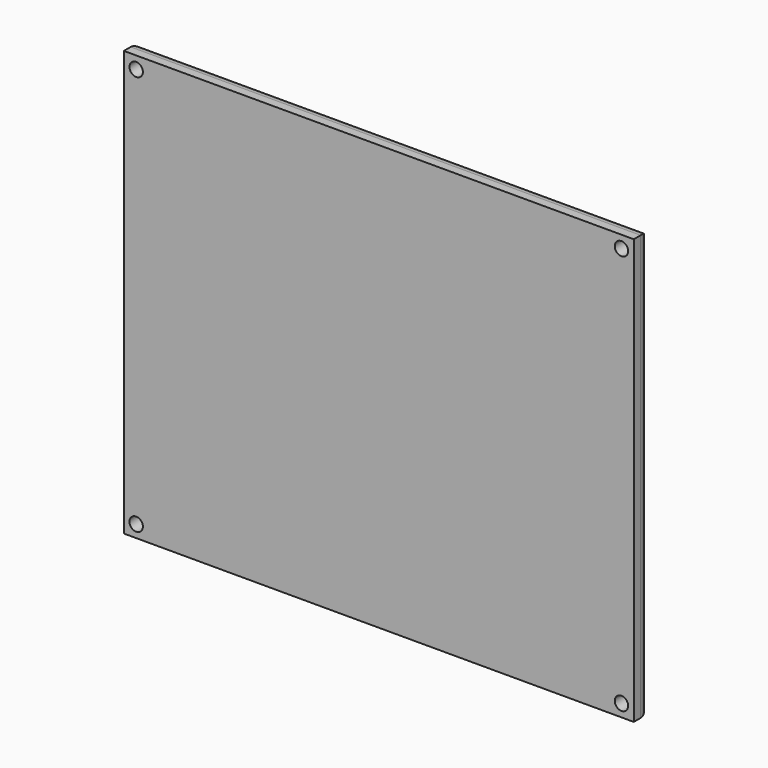
from build123d import *

# Parameters (mm, degrees)
F0_W           = 120
F0_H           = 100
F1_DEPTH       = 5
F2_D           = 3.15
F2_CSINK_D     = 5
F2_CSINK_ANGLE = 90
F3_T1_DEPTH    = 135
F3_T3_DEPTH    = 115


# Not quite as in the source:
# - a fillet or chamfer that OpenCascade refuses, or shapes differently, is made with other operations: its cross-section is extruded or revolved along the edge and cut away or added


with BuildPart() as f1:
    # F0 (on Front) → F1 (new body)
    with BuildSketch(Plane.XZ):
        with Locations((-0.298661174, 0)):
            Rectangle(F0_W, F0_H)
    extrude(amount=F1_DEPTH)

    # F2 (through all)
    with Locations(Plane(origin=(0, 0, 0), x_dir=(1, 0, 0), z_dir=(0, 1, 0))):
        with Locations((-57.398661174, -47.1), (56.801338826, -47.1), (56.801338826, 47.1), (-57.398661174, 47.1)):
            CounterSinkHole(F2_D / 2, F2_CSINK_D / 2, counter_sink_angle=F2_CSINK_ANGLE)

    # F3: fillet of radius 3 on 4 edges, made by hand

    # F3_s2 → F3_t1 (cut)
    with BuildSketch(Plane.YZ.offset(-67.798661174)):
        with BuildLine():
            ThreePointArc((0, -47), (-0.8786796564, -49.1213203436), (-3, -50))
            Line((-3, -50), (0, -50))
            Line((0, -50), (0, -47))
        make_face()
        with BuildLine():
            ThreePointArc((-3, 50), (-0.8786796564, 49.1213203436), (0, 47))
            Line((0, 47), (0, 50))
            Line((0, 50), (-3, 50))
        make_face()
    extrude(amount=F3_T1_DEPTH, mode=Mode.SUBTRACT)

    # F3_s4 → F3_t3 (cut)
    with BuildSketch(Plane.XY.offset(-57.5)):
        with BuildLine():
            ThreePointArc((59.701338826, -3), (58.8226591695, -0.8786796564), (56.701338826, 0))
            Line((56.701338826, 0), (59.701338826, 0))
            Line((59.701338826, 0), (59.701338826, -3))
        make_face()
        with BuildLine():
            ThreePointArc((-60.298661174, -3), (-59.4199815176, -0.8786796564), (-57.298661174, 0))
            Line((-57.298661174, 0), (-60.298661174, 0))
            Line((-60.298661174, 0), (-60.298661174, -3))
        make_face()
    extrude(amount=F3_T3_DEPTH, mode=Mode.SUBTRACT)


solid = f1.part
